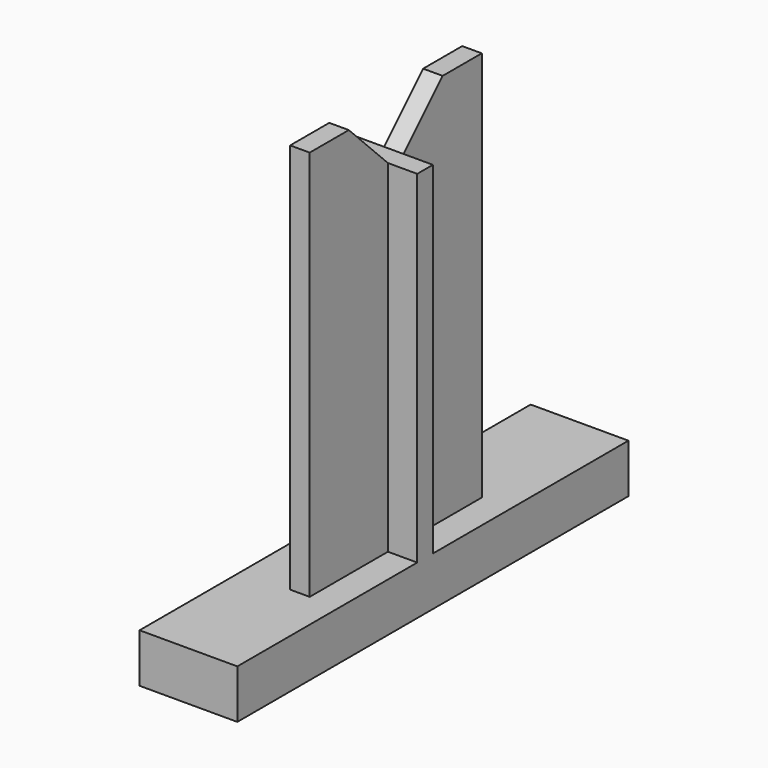
from build123d import *

# Parameters (mm, degrees)
F0_W     = 10
F0_H     = 50
F1_DEPTH = 5
F2_W     = 10
F2_H     = 2
F3_DEPTH = 35
F4_W     = 2
F4_H     = 10
F5_DEPTH = 40
F6_W     = 2
F6_H     = 10
F7_DEPTH = 40
F8_SIZE  = 5
F9_SIZE  = 4.99999


# Not quite as in the source:
# - a fillet or chamfer is up to 0.001 mm smaller than in the source, because OpenCascade refuses the exact size


with BuildPart() as f1:
    # F0 (on Top) → F1 (new body)
    with BuildSketch(Plane.XY):
        with Locations((-41.2431620061, 9.2969734803)):
            Rectangle(F0_W, F0_H)
    extrude(amount=F1_DEPTH)

    # F2 (on face) → F3 (join)
    with BuildSketch(Plane.XY.offset(5)):
        with Locations((-41.2431620061, 8.2969734803)):
            Rectangle(F2_W, F2_H)
    extrude(amount=F3_DEPTH)

    # F6 (on face) → F7 (join)
    with BuildSketch(Plane.XY.offset(5)):
        with Locations((-40.2431620061, 14.2969734803)):
            Rectangle(F6_W, F6_H)
    extrude(amount=F7_DEPTH)

    # F9 (size 5 in the source; OpenCascade refuses exactly that, so slightly less here)
    f9_edges = [f1.edges().sort_by_distance(p)[0] for p in [
        (-40.243162, 9.296973, 45),
    ]]
    chamfer(f9_edges, length=F9_SIZE)


with BuildPart() as f5:
    # F4 (on face) → F5 (new body)
    with BuildSketch(Plane.XY.offset(5)):
        with Locations((-40.2431620061, 2.2969734803)):
            Rectangle(F4_W, F4_H)
    extrude(amount=F5_DEPTH)

    # F8
    f8_edges = [f5.edges().sort_by_distance(p)[0] for p in [
        (-40.243162, 7.296973, 45),
    ]]
    chamfer(f8_edges, length=F8_SIZE)


solid = Compound([f1.part, f5.part])
